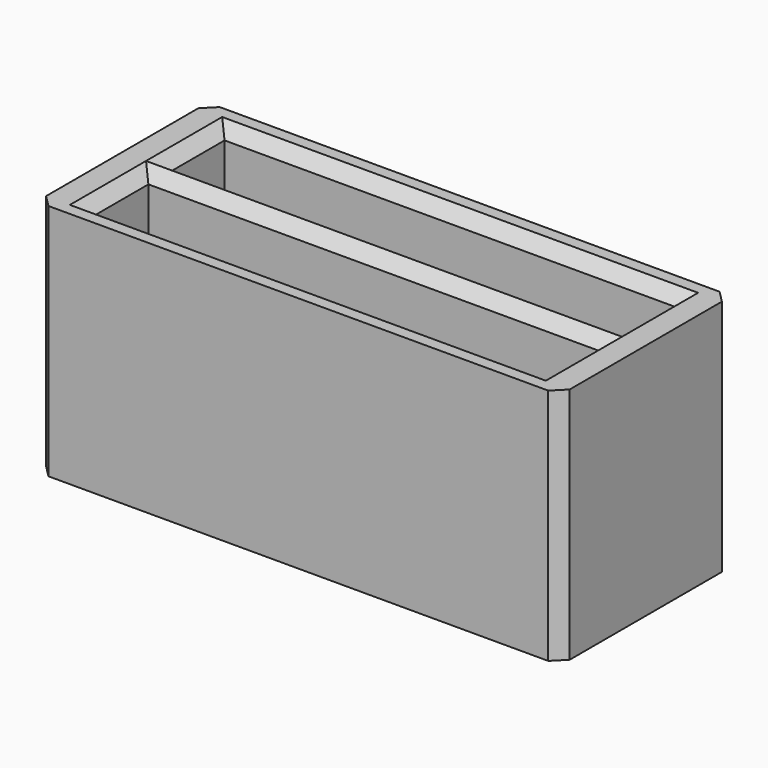
from build123d import *

# Parameters (mm, degrees)
F0_W         = 19
F0_H         = 3
F1_DEPTH     = 10
F2_SIZE      = 0.5
F3_SIZE      = 0.49999
F4_SIZE      = 0.49999
F5_TEXT_SIZE = 6.2323497906
F6_DEPTH     = 0.5


# Not quite as in the source:
# - a fillet or chamfer is up to 0.001 mm smaller than in the source, because OpenCascade refuses the exact size
# - Text() gives the source's letters only with a copy of the font that has no kerning and outlines rounded to 1/6400 em; it was checked with that copy


with BuildPart() as f1:
    # F0 (on Top) → F1 (new body)
    with BuildSketch(Plane.XY):
        Polygon((-13.0745237693, 0), (-11.5745237693, 0), (7.4254762307, 0), (7.9254762307, 0), (8.9254762307, 0), (8.9254762307, 4), (8.9254762307, 5), (8.9254762307, 9), (-13.0745237693, 9), (-13.0745237693, 5), (-13.0745237693, 4), align=None)
        with Locations((-2.0745237693, 2.5)):
            Rectangle(F0_W, F0_H, mode=Mode.SUBTRACT)
        with Locations((-2.0745237693, 6.5)):
            Rectangle(F0_W, F0_H, mode=Mode.SUBTRACT)
    extrude(amount=F1_DEPTH)

    # F2
    f2_edges = [f1.edges().sort_by_distance(p)[0] for p in [
        (-13.074524, 9, 5),
        (-13.074524, 0, 5),
        (8.925476, 9, 5),
        (8.925476, 0, 5),
    ]]
    chamfer(f2_edges, length=F2_SIZE)

    # F3 (size 0.5 in the source; OpenCascade refuses exactly that, so slightly less here)
    f3_edges = [f1.edges().sort_by_distance(p)[0] for p in [
        (-2.074524, 8, 10),
        (-11.574524, 6.5, 10),
        (-2.074524, 5, 10),
        (7.425476, 6.5, 10),
        (7.425476, 2.5, 10),
        (-2.074524, 4, 10),
        (-2.074524, 1, 10),
        (-11.574524, 2.5, 10),
    ]]
    chamfer(f3_edges, length=F3_SIZE)

    # F4 (size 0.5 in the source; OpenCascade refuses exactly that, so slightly less here)
    f4_edges = [f1.edges().sort_by_distance(p)[0] for p in [
        (-2.074524, 8, 0),
        (7.425476, 6.5, 0),
        (-2.074524, 5, 0),
        (-11.574524, 6.5, 0),
        (-11.574524, 2.5, 0),
        (-2.074524, 4, 0),
        (7.425476, 2.5, 0),
        (-2.074524, 1, 0),
    ]]
    chamfer(f4_edges, length=F4_SIZE)

    # F5 (on face) → F6 (cut)
    with BuildSketch(Plane(origin=(0, 9, 0), x_dir=(-1, 0, 0), z_dir=(0, 1, 0))):
        with Locations((-7.9941827699, 2.7914835374)):
            Text('DHBW', F5_TEXT_SIZE, font='Open Sans', font_style=FontStyle.BOLD, text_align=(TextAlign.LEFT, TextAlign.BOTTOM))
    extrude(amount=-F6_DEPTH, mode=Mode.SUBTRACT)


solid = f1.part
